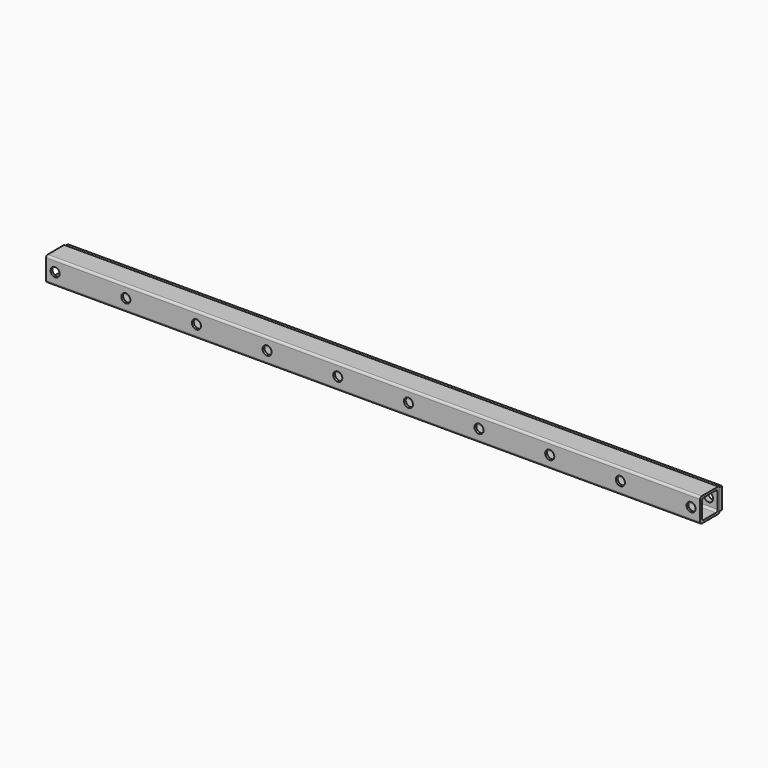
from build123d import *

# Parameters (mm, degrees)
F1_DEPTH = 2743.2
F2_W     = 12.7
F2_H     = 88.9
F3_DEPTH = 2743.2
F4_R     = 19.05
F5_DEPTH = 114.301
F6_R     = 19.05
F7_DEPTH = 254


# Not quite as in the source:
# - a feature names something its author has since deleted; it is built from what else it names


with BuildPart() as f1:
    # F0 (on Right) → F1 (new body)
    with BuildSketch(Plane.YZ):
        with BuildLine():
            Line((-92.71, 0), (-8.89, 0))
            ThreePointArc((-8.89, 0), (-2.6038207153, 2.6038207153), (0, 8.89))
            Line((0, 8.89), (0, 92.71))
            ThreePointArc((0, 92.71), (-2.6038207153, 98.9961792847), (-8.89, 101.6))
            Line((-8.89, 101.6), (-92.71, 101.6))
            ThreePointArc((-92.71, 101.6), (-98.9961792847, 98.9961792847), (-101.6, 92.71))
            Line((-101.6, 92.71), (-101.6, 8.89))
            ThreePointArc((-101.6, 8.89), (-98.9961792847, 2.6038207153), (-92.71, 0))
        make_face()
        with BuildLine():
            Line((-83.185, 92.075), (-18.415, 92.075))
            ThreePointArc((-18.415, 92.075), (-12.1288207153, 89.4711792847), (-9.525, 83.185))
            Line((-9.525, 83.185), (-9.525, 18.415))
            ThreePointArc((-9.525, 18.415), (-12.1288207153, 12.1288207153), (-18.415, 9.525))
            Line((-18.415, 9.525), (-83.185, 9.525))
            ThreePointArc((-83.185, 9.525), (-89.4711792847, 12.1288207153), (-92.075, 18.415))
            Line((-92.075, 18.415), (-92.075, 83.185))
            ThreePointArc((-92.075, 83.185), (-89.4711792847, 89.4711792847), (-83.185, 92.075))
        make_face(mode=Mode.SUBTRACT)
    extrude(amount=-F1_DEPTH)


with BuildPart() as f3:
    # F2 (on Right) → F3 (new body)
    with BuildSketch(Plane.YZ):
        with Locations((6.35, 51.8165992945)):
            Rectangle(F2_W, F2_H)
    extrude(amount=-F3_DEPTH)


with BuildPart() as f5_tool:
    # F4 (on face) → F5 (new body, through all)
    with BuildSketch(Plane(origin=(0, 12.7, 0), x_dir=(-1, 0, 0), z_dir=(0, 1, 0))):
        with Locations((38.1, 51.8165992945)):
            Circle(F4_R)
        with Locations((334.4418, 51.8165992945)):
            Circle(F4_R)
        with Locations((630.7836, 51.8165992945)):
            Circle(F4_R)
        with Locations((927.1254, 51.8165992945)):
            Circle(F4_R)
        with Locations((1223.4672, 51.8165992945)):
            Circle(F4_R)
        with Locations((1519.809, 51.8165992945)):
            Circle(F4_R)
        with Locations((1816.1508, 51.8165992945)):
            Circle(F4_R)
        with Locations((2112.4926, 51.8165992945)):
            Circle(F4_R)
        with Locations((2408.8344, 51.8165992945)):
            Circle(F4_R)
        with Locations((2705.1762, 51.8165992945)):
            Circle(F4_R)
    extrude(amount=-F5_DEPTH)


with BuildPart() as f1_1:
    add(f1.part)

    # F5: cut by f5_tool
    add(f5_tool.part, mode=Mode.SUBTRACT)

    # F6 (on face) → F7 (cut)
    with BuildSketch(Plane.XZ.offset(101.6)):
        with Locations((-38.1, 51.8165992945)):
            Circle(F6_R)
        with Locations((-334.4418, 51.8165992945)):
            Circle(F6_R)
        with Locations((-630.7836, 51.8165992945)):
            Circle(F6_R)
        with Locations((-927.1254, 51.8165992945)):
            Circle(F6_R)
        with Locations((-1223.4672, 51.8165992945)):
            Circle(F6_R)
        with Locations((-1519.809, 51.8165992945)):
            Circle(F6_R)
        with Locations((-1816.1508, 51.8165992945)):
            Circle(F6_R)
        with Locations((-2112.4926, 51.8165992945)):
            Circle(F6_R)
        with Locations((-2408.8344, 51.8165992945)):
            Circle(F6_R)
        with BuildLine():
            ThreePointArc((-2705.1381000001, 32.7666373946), (-2691.6923521627, 38.359692239), (-2686.1262, 51.8165992945))
            ThreePointArc((-2686.1262, 51.8165992945), (-2691.6923521626, 65.27350635), (-2705.1380999999, 70.8665611945))
            ThreePointArc((-2705.1380999999, 70.8665611945), (-2724.15, 51.8165992947), (-2705.1381000001, 32.7666373946))
        make_face()
        with BuildLine():
            ThreePointArc((-2705.1380999999, 70.8665611945), (-2691.6923521626, 65.27350635), (-2686.1262, 51.8165992945))
            ThreePointArc((-2686.1262, 51.8165992945), (-2691.6923521627, 38.359692239), (-2705.1381000001, 32.7666373946))
            ThreePointArc((-2705.1381000001, 32.7666373946), (-2691.6430929446, 38.3327514572), (-2686.05, 51.8165992945))
            ThreePointArc((-2686.05, 51.8165992945), (-2691.6430929445, 65.3004471318), (-2705.1380999999, 70.8665611945))
        make_face()
        with BuildLine():
            ThreePointArc((-2705.1381000001, 32.7666373946), (-2724.15, 51.8165992947), (-2705.1380999999, 70.8665611945))
            ThreePointArc((-2705.1380999999, 70.8665611945), (-2724.2262, 51.8165992947), (-2705.1381000001, 32.7666373946))
        make_face()
    extrude(amount=-F7_DEPTH, mode=Mode.SUBTRACT)


with BuildPart() as f3_1:
    add(f3.part)

    # F5: cut by f5_tool
    add(f5_tool.part, mode=Mode.SUBTRACT)


solid = Compound([f1_1.part, f3_1.part])
